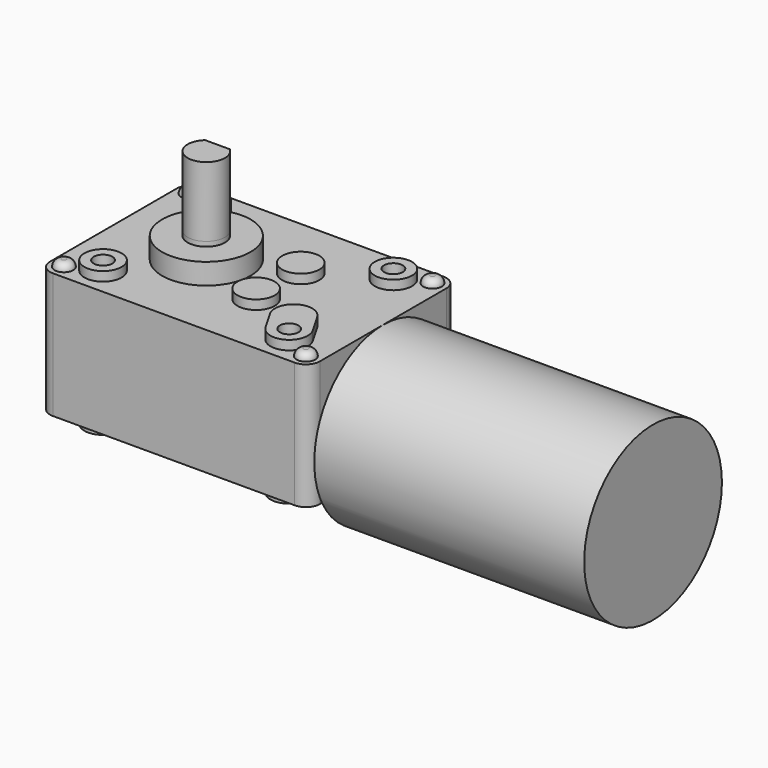
from build123d import *

# Parameters (mm, degrees)
F1_DEPTH  = 27
F2_R      = 4
F3_DEPTH  = 2
F4_DEPTH  = 29
F5_R      = 9.5
F6_DEPTH  = 4.5
F7_DEPTH  = 31.5
F8_R      = 4
F9_DEPTH  = 1
F11_DEPTH = 15
F12_R     = 4
F13_DEPTH = 0.1
F14_R     = 18.5
F15_DEPTH = 58
F16_R     = 2
F17_DEPTH = 1.5
F18_R     = 1.49999
F19_R     = 2
F20_DEPTH = 5
F21_R     = 2
F22_DEPTH = 5


# Not quite as in the source:
# - a fillet or chamfer is up to 0.001 mm smaller than in the source, because OpenCascade refuses the exact size


with BuildPart() as f1:
    # F0 (on Top) → F1 (new body)
    with BuildSketch(Plane.XY):
        with BuildLine():
            ThreePointArc((38, 17), (37.1213203436, 19.1213203436), (35, 20))
            Line((35, 20), (-17, 20))
            ThreePointArc((-17, 20), (-19.1213203436, 19.1213203436), (-20, 17))
            Line((-20, 17), (-20, -17))
            ThreePointArc((-20, -17), (-19.1213203436, -19.1213203436), (-17, -20))
            Line((-17, -20), (35, -20))
            ThreePointArc((35, -20), (37.1213203436, -19.1213203436), (38, -17))
            Line((38, -17), (38, 17))
        make_face()
    extrude(amount=F1_DEPTH)

    # F2 (on face) → F3 (join)
    with BuildSketch(Plane.XY.offset(27)):
        with Locations((-11, 14)):
            Circle(F2_R)
        with Locations((29, 14)):
            Circle(F2_R)
        with Locations((-11, -14)):
            Circle(F2_R)
        with BuildLine():
            Line((32.4641016151, -12), (29.9641016151, -7.6698729811))
            ThreePointArc((29.9641016151, -7.6698729811), (24.5, -6.2057713659), (23.0358983849, -11.6698729811))
            Line((23.0358983849, -11.6698729811), (25.5358983849, -16))
            ThreePointArc((25.5358983849, -16), (31, -17.4641016151), (32.4641016151, -12))
        make_face()
        with Locations((15.5, 6)):
            Circle(F2_R)
        with Locations((15.5, -6)):
            Circle(F2_R)
    extrude(amount=F3_DEPTH)

    # F2 (on face) → F4 (join)
    with BuildSketch(Plane.XY.offset(27)):
        with Locations((-11, 14)):
            Circle(F2_R)
        with Locations((29, 14)):
            Circle(F2_R)
        with Locations((-11, -14)):
            Circle(F2_R)
        with BuildLine():
            Line((32.4641016151, -12), (29.9641016151, -7.6698729811))
            ThreePointArc((29.9641016151, -7.6698729811), (24.5, -6.2057713659), (23.0358983849, -11.6698729811))
            Line((23.0358983849, -11.6698729811), (25.5358983849, -16))
            ThreePointArc((25.5358983849, -16), (31, -17.4641016151), (32.4641016151, -12))
        make_face()
        with Locations((15.5, 6)):
            Circle(F2_R)
        with Locations((15.5, -6)):
            Circle(F2_R)
    extrude(amount=-F4_DEPTH)

    # F5 (on face) → F6 (join)
    with BuildSketch(Plane.XY.offset(27)):
        Circle(F5_R)
    extrude(amount=F6_DEPTH)

    # F5 (on face) → F7 (join)
    with BuildSketch(Plane.XY.offset(27)):
        Circle(F5_R)
    extrude(amount=-F7_DEPTH)

    # F8 (on face) → F9 (join)
    with BuildSketch(Plane.XY.offset(31.5)):
        Circle(F8_R)
    extrude(amount=F9_DEPTH)

    # F10 (on face) → F11 (join)
    with BuildSketch(Plane.XY.offset(32.5)):
        with BuildLine():
            Line((2.6457513111, 3), (-2.6457513111, 3))
            ThreePointArc((-2.6457513111, 3), (0, -4), (2.6457513111, 3))
        make_face()
    extrude(amount=F11_DEPTH)

    # F12 (on face) → F13 (cut)
    with BuildSketch(Plane(origin=(0, 0, -4.5), x_dir=(1, 0, 0), z_dir=(0, 0, -1))):
        Circle(F12_R)
    extrude(amount=-F13_DEPTH, mode=Mode.SUBTRACT)

    # F14 (on face) → F15 (join)
    with BuildSketch(Plane.YZ.offset(38)):
        with Locations((0, 8.5)):
            Circle(F14_R)
    extrude(amount=F15_DEPTH)

    # F16 (on face) → F17 (join)
    with BuildSketch(Plane.XY.offset(27)):
        with Locations((-17, 17)):
            Circle(F16_R)
        with Locations((35, 17)):
            Circle(F16_R)
        with Locations((35, -17)):
            Circle(F16_R)
        with Locations((-17, -17)):
            Circle(F16_R)
    extrude(amount=F17_DEPTH)

    # F18 (radius 1.5 in the source; OpenCascade refuses exactly that, so slightly less here)
    f18_edges = [f1.edges().sort_by_distance(p)[0] for p in [
        (-19, 17, 28.5),
        (-19, -17, 28.5),
        (33, -17, 28.5),
        (33, 17, 28.5),
    ]]
    fillet(f18_edges, radius=F18_R)

    # F19 (on face) → F20 (cut)
    with BuildSketch(Plane.XY.offset(29)):
        with Locations((-11, 14)):
            Circle(F19_R)
        with Locations((-11, -14)):
            Circle(F19_R)
        with Locations((29, -14)):
            Circle(F19_R)
        with Locations((29, 14)):
            Circle(F19_R)
    extrude(amount=-F20_DEPTH, mode=Mode.SUBTRACT)

    # F21 (on face) → F22 (cut)
    with BuildSketch(Plane(origin=(0, 0, -2), x_dir=(1, 0, 0), z_dir=(0, 0, -1))):
        with Locations((29, 14)):
            Circle(F21_R)
        with Locations((29, -14)):
            Circle(F21_R)
        with Locations((-11, -14)):
            Circle(F21_R)
        with Locations((-11, 14)):
            Circle(F21_R)
    extrude(amount=-F22_DEPTH, mode=Mode.SUBTRACT)


solid = f1.part
